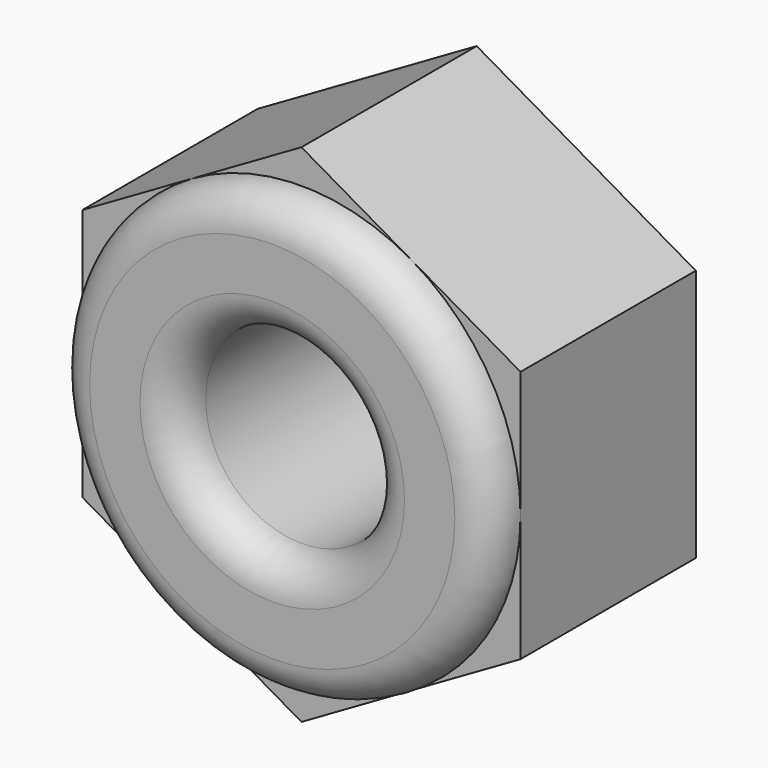
from build123d import *

# Parameters (mm, degrees)
F0_R     = 2.0828
F1_DEPTH = 4.7625
F2_R     = 4.7625
F2_R_2   = 2.0828
F3_DEPTH = 0.79375
F4_R     = 0.79374
F5_R     = 0.79375


# Not quite as in the source:
# - a fillet or chamfer is up to 0.001 mm smaller than in the source, because OpenCascade refuses the exact size


with BuildPart() as f1:
    # F0 (on Front) → F1 (new body)
    with BuildSketch(Plane.XZ):
        Polygon((4.7625, -2.749630657), (4.7625, 2.749630657), (0, 5.499261314), (-4.7625, 2.749630657), (-4.7625, -2.749630657), (0, -5.499261314), align=None)
        Circle(F0_R, mode=Mode.SUBTRACT)
    extrude(amount=-F1_DEPTH)

    # F2 (on face) → F3 (join)
    with BuildSketch(Plane.XZ):
        Circle(F2_R)
        Circle(F2_R_2, mode=Mode.SUBTRACT)
    extrude(amount=F3_DEPTH)

    # F4 (radius 0.79375 in the source; OpenCascade refuses exactly that, so slightly less here)
    f4_edges = [f1.edges().sort_by_distance(p)[0] for p in [
        (-4.7625, -0.79375, 0),
        (-2.0828, -0.79375, 0),
    ]]
    fillet(f4_edges, radius=F4_R)

    # F5
    f5_edges = [f1.edges().sort_by_distance(p)[0] for p in [
        (-2.0828, 4.7625, 0),
    ]]
    fillet(f5_edges, radius=F5_R)


solid = f1.part
